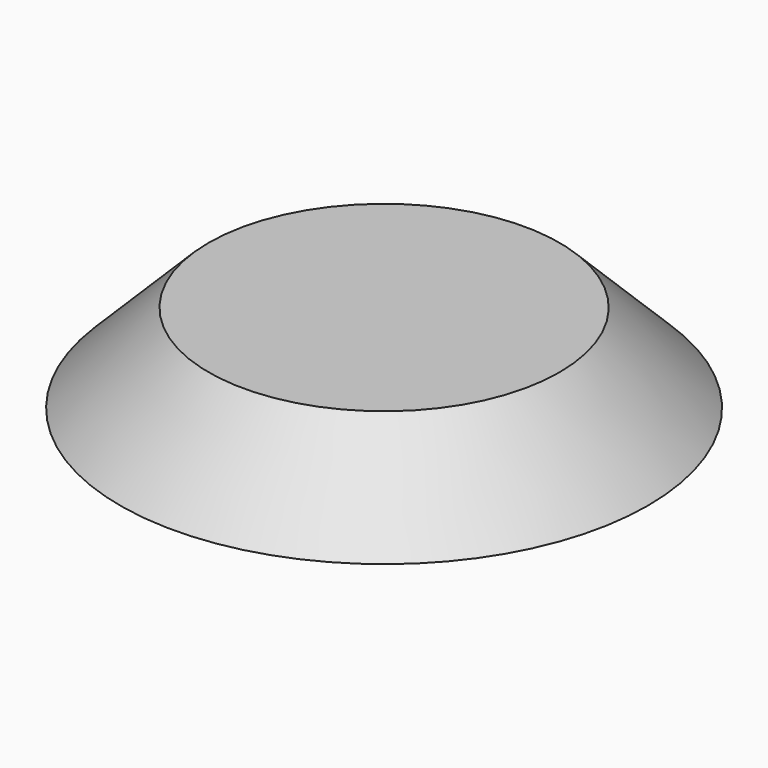
from build123d import *

# Parameters (mm, degrees)
F0_R     = 75.7334289918
F1_DEPTH = 25.4
F1_TAPER = 45


with BuildPart() as f1:
    # F0 (on Top) → F1 (new body)
    with BuildSketch(Plane.XY):
        Circle(F0_R)
    extrude(amount=F1_DEPTH, taper=F1_TAPER)


solid = f1.part
